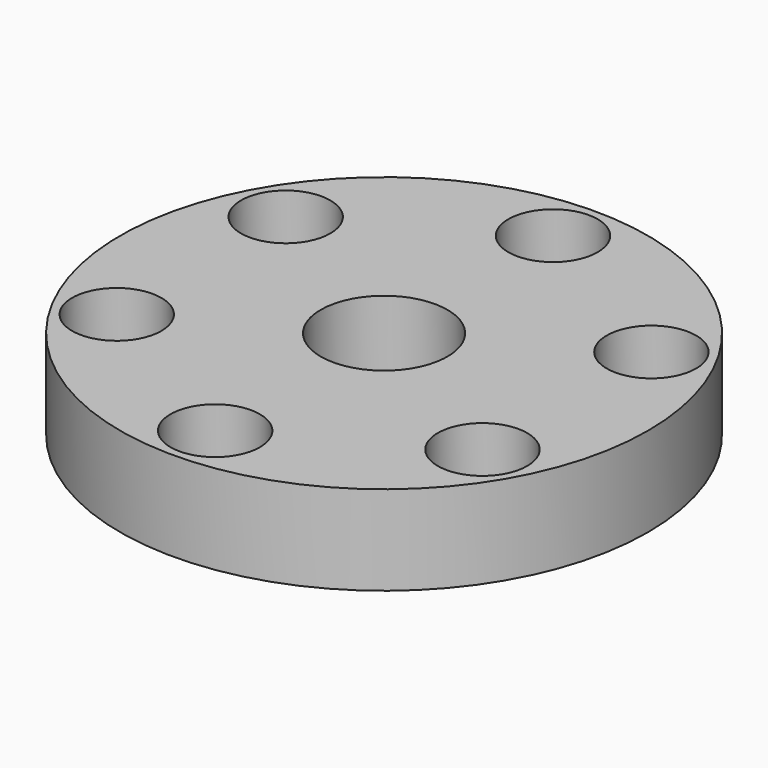
from build123d import *

# Parameters (mm, degrees)
F0_R           = 37.5
F1_DEPTH       = 12.7
F3_D           = 18
F5_D           = 6.5
F5_CBORE_D     = 12.7
F5_CBORE_DEPTH = 10


# Not quite as in the source:
# - a length typed as a fraction of an inch, garbled in the dataset ("3 / 203.2 mm" for 3/8 in), is restored


with BuildPart() as f1:
    # F0 (on Top) → F1 (new body)
    with BuildSketch(Plane.XY):
        Circle(F0_R)
    extrude(amount=F1_DEPTH)

    # F3 (through all)
    with Locations(Plane.XY.offset(12.7)):
        with Locations((0, 0)):
            Hole(F3_D / 2)

    # F5 (through all)
    with Locations(Plane.XY.offset(12.7)):
        with Locations((0, 30), (25.9807621135, 15), (25.9807621135, -15), (0, -30), (-25.9807621135, -15), (-25.9807621135, 15)):
            CounterBoreHole(F5_D / 2, F5_CBORE_D / 2, F5_CBORE_DEPTH)


solid = f1.part
